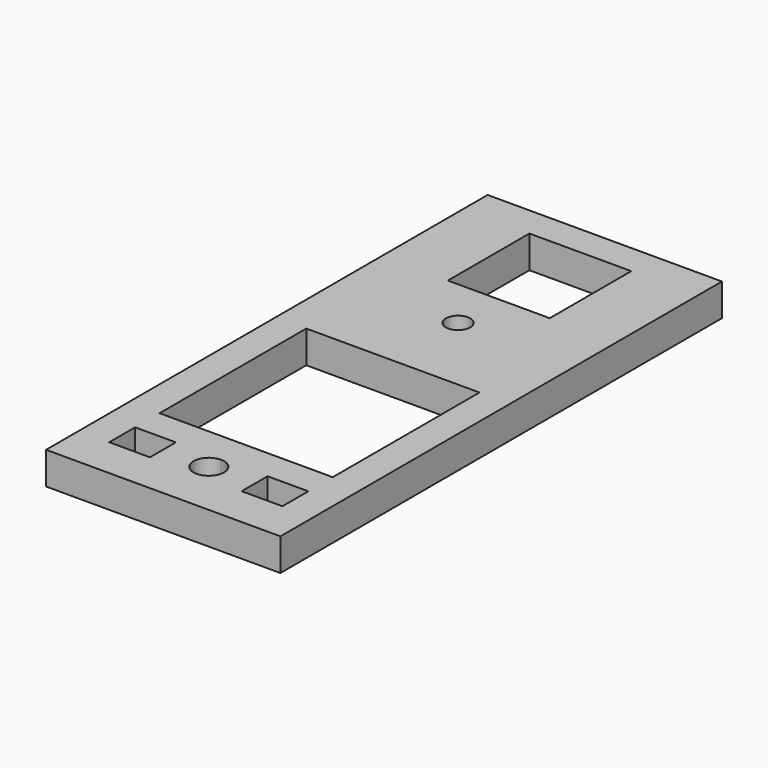
from build123d import *

# Parameters (mm, degrees)
F0_W     = 23
F0_H     = 54.175
F0_W_2   = 4
F0_H_2   = 3.175
F0_W_3   = 17
F0_H_3   = 18
F0_W_4   = 10
F0_H_4   = 10
F0_R     = 1.2
F1_DEPTH = 3.175


# Not quite as in the source:
# - a length typed as a fraction of an inch, garbled in the dataset ("3 / 203.2 mm" for 3/8 in), is restored
# - a feature names something its author has since deleted; it is built from what else it names


with BuildPart() as f1:
    # F0 (on Top) → F1 (new body)
    with BuildSketch(Plane.XY):
        with Locations((11.4247928681, 25.3005515426)):
            Rectangle(F0_W, F0_H)
        with Locations((4.9247928681, 3.8005515426)):
            Rectangle(F0_W_2, F0_H_2, mode=Mode.SUBTRACT)
        with BuildLine():
            ThreePointArc((11.4247928681, 5.3005515426), (12.4854530398, 4.8612117144), (12.9247928681, 3.8005515426))
            ThreePointArc((12.9247928681, 3.8005515426), (10.3641326963, 2.7398913709), (11.4247928681, 5.3005515426))
        make_face(mode=Mode.SUBTRACT)
        with Locations((17.9247928681, 3.8005515426)):
            Rectangle(F0_W_2, F0_H_2, mode=Mode.SUBTRACT)
        with Locations((11.4247928681, 17.3880515426)):
            Rectangle(F0_W_3, F0_H_3, mode=Mode.SUBTRACT)
        Polygon((6.4247928681, 29.3880515426), (6.4247928681, 39.3880515426), (6.4247928681, 49.3880515426), (16.4247928681, 49.3880515426), (16.4247928681, 39.3880515426), (16.4247928681, 29.3880515426), align=None, mode=Mode.SUBTRACT)
        with Locations((11.4247928681, 34.3880515426)):
            Rectangle(F0_W_4, F0_H_4)
        with Locations((11.4247928681, 34.3880515426)):
            Circle(F0_R, mode=Mode.SUBTRACT)
    extrude(amount=F1_DEPTH)


solid = f1.part
